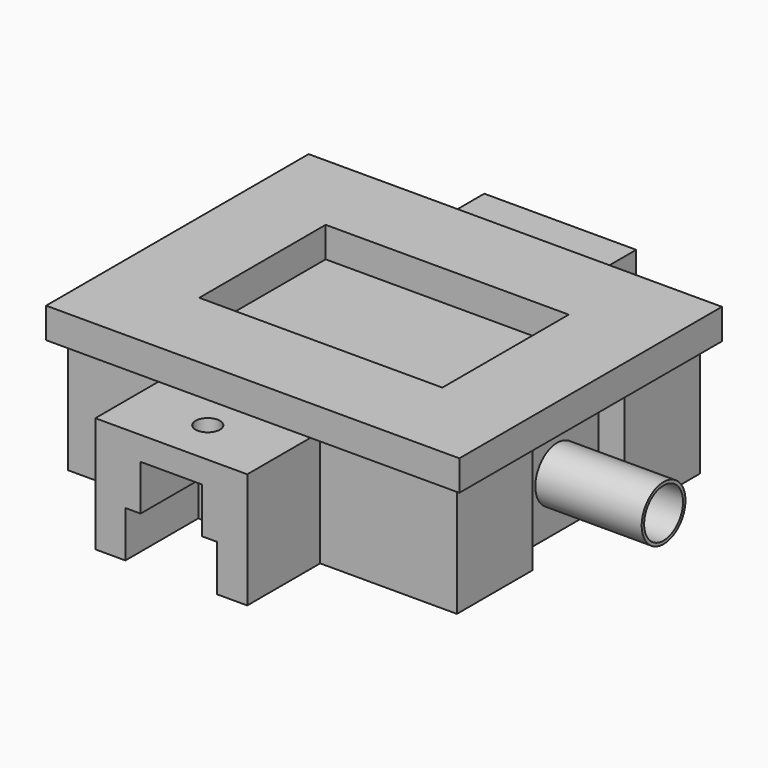
from build123d import *

# Parameters (mm, degrees)
F0_W      = 54
F0_H      = 19
F1_DEPTH  = 20
F2_R      = 4.5
F3_DEPTH  = 1.5
F4_DEPTH  = 19
F5_T      = -0.5
F6_W      = 64
F6_H      = 50
F6_W_2    = 54
F6_H_2    = 40
F7_DEPTH  = 19
F9_DEPTH  = 25
F11_W     = 68
F11_H     = 54
F11_W_2   = 64
F11_H_2   = 50
F12_DEPTH = 5
F11_W_3   = 54
F11_H_3   = 40
F11_W_4   = 40
F11_H_4   = 26
F15_DEPTH = 15
F16_R     = 2
F17_DEPTH = 8.901


with BuildPart() as f1:
    # F0 (on Front) → F1 (new body, symmetric)
    with BuildSketch(Plane.XZ):
        with Locations((3, 9.5)):
            Rectangle(F0_W, F0_H)
    extrude(amount=F1_DEPTH, both=True)

    # F2 (on face) → F3 (join)
    with BuildSketch(Plane.YZ.offset(30)):
        Polygon((-8.5, 17.5), (-8.5, 0.5), (0, 0.5), (8.5, 0.5), (8.5, 17.5), (0, 17.5), align=None)
        with Locations((0, 9)):
            Circle(F2_R, mode=Mode.SUBTRACT)
    extrude(amount=F3_DEPTH)

    # F4 (add): a face of the model
    f4_faces = [f1.faces().sort_by_distance(p)[0] for p in [
        (30, 0, 9),
    ]]
    extrude(f4_faces, amount=F4_DEPTH)

    # F5
    f5_openings = [f1.faces().sort_by_distance(p)[0] for p in [
        (49, 0, 9),
    ]]
    offset(amount=F5_T, openings=f5_openings, kind=Kind.INTERSECTION)


with BuildPart() as f7:
    # F6 (on face) → F7 (new body, through all)
    with BuildSketch(Plane.XY.offset(19)):
        with Locations((3, 0)):
            Rectangle(F6_W, F6_H)
        with Locations((3, 0)):
            Rectangle(F6_W_2, F6_H_2, mode=Mode.SUBTRACT)
    extrude(amount=-F7_DEPTH)

    # F8 (on face) → F9 (cut)
    with BuildSketch(Plane.YZ.offset(35)):
        Polygon((0, -0.5), (9.5, -0.5), (9.5, 19), (0, 19), (-9.5, 19), (-9.5, -0.5), align=None)
    extrude(amount=-F9_DEPTH, mode=Mode.SUBTRACT)

    # F13 (on face) → F15 (join)
    with BuildSketch(Plane(origin=(0, 25, 0), x_dir=(-1, 0, 0), z_dir=(0, 1, 0))):
        Polygon((-12.5, 0), (-7.55, 0), (-7.55, 7.6), (-5.05, 7.6), (-5.05, 15.1), (0, 15.1), (5.05, 15.1), (5.05, 7.6), (7.55, 7.6), (7.55, 0), (12.5, 0), (12.5, 19), (0, 19), (-12.5, 19), align=None)
    extrude(amount=F15_DEPTH)

    # F16 (on face) → F17 (cut, through all)
    with BuildSketch(Plane(origin=(0, 0, 15.1), x_dir=(1, 0, 0), z_dir=(0, 0, -1))):
        with Locations((0, -32.5)):
            Circle(F16_R)
    extrude(amount=-F17_DEPTH, mode=Mode.SUBTRACT)

    # F18: F7 across plane


with BuildPart() as f12:
    # F11 (on face) → F12 (new body)
    with BuildSketch(Plane.XY.offset(19)):
        with Locations((3, 0)):
            Rectangle(F11_W, F11_H)
        with Locations((3, 0)):
            Rectangle(F11_W_2, F11_H_2, mode=Mode.SUBTRACT)
    extrude(amount=F12_DEPTH)



with BuildPart() as f12b:
    # F11 (on face) → F12, piece 2 (new body)
    with BuildSketch(Plane.XY.offset(19)):
        with Locations((3, 0)):
            Rectangle(F11_W_3, F11_H_3)
        with Locations((3, 0)):
            Rectangle(F11_W_4, F11_H_4, mode=Mode.SUBTRACT)
    extrude(amount=F12_DEPTH)


with BuildPart() as f12_1:
    add(f12.part)

    add(f12b.part)  # F12#3 merges F12b
    # F6 (on face) → F12, piece 3 (join)
    with BuildSketch(Plane.XY.offset(19)):
        with Locations((3, 0)):
            Rectangle(F6_W, F6_H)
        with Locations((3, 0)):
            Rectangle(F6_W_2, F6_H_2, mode=Mode.SUBTRACT)
    extrude(amount=F12_DEPTH)


with BuildPart() as f7_1:
    add(f7.part)
    add(f7.part.mirror(Plane.XZ))


solid = Compound([f1.part, f12_1.part, f7_1.part])
